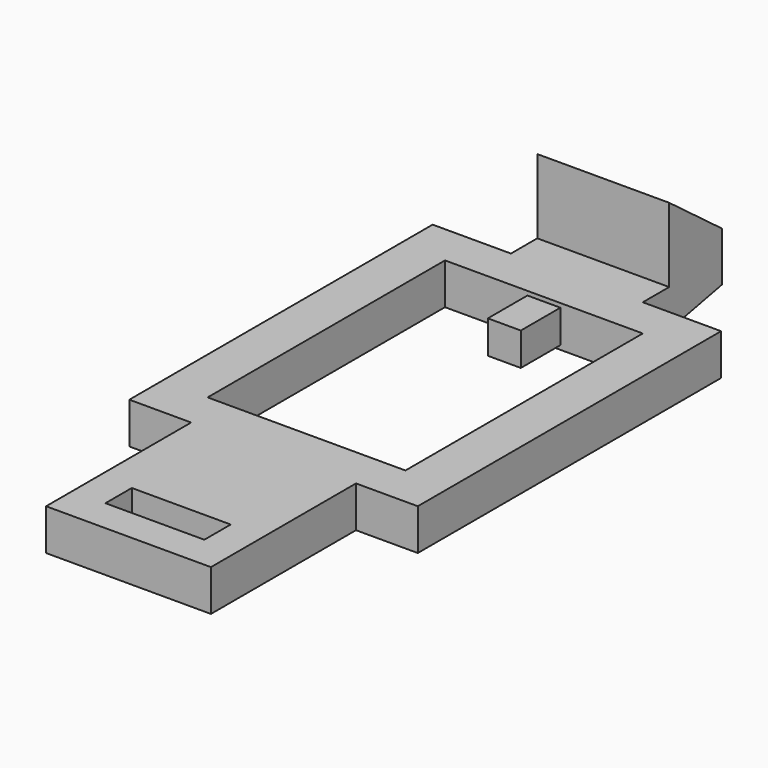
from build123d import *

# Parameters (mm, degrees)
F0_W     = 6
F0_H     = 2
F1_DEPTH = 2.5
F2_W     = 8
F2_H     = 4
F3_DEPTH = 4.5
F4_SIZE2 = 3.99999
F4_SIZE  = 2.99999
F5_SIZE2 = 1
F5_SIZE  = 5
F6_W     = 2
F6_H     = 3
F7_DEPTH = 0.25
F8_W     = 2
F8_H     = 3
F9_DEPTH = 0.25


# Not quite as in the source:
# - a fillet or chamfer is up to 0.001 mm smaller than in the source, because OpenCascade refuses the exact size


with BuildPart() as f1:
    # F0 (on Top) → F1 (new body)
    with BuildSketch(Plane.XY):
        Polygon((-5, 11), (-5, 0), (5, 0), (5, 11), (8.75, 11), (8.75, 34), (4, 34), (4, 40), (-4, 40), (-4, 34), (-8.75, 34), (-8.75, 11), align=None)
        with Locations((0, 3)):
            Rectangle(F0_W, F0_H, mode=Mode.SUBTRACT)
        Polygon((-6, 13.5), (-6, 31.5), (-1, 31.5), (-1, 28.5), (1, 28.5), (1, 31.5), (6, 31.5), (6, 13.5), align=None, mode=Mode.SUBTRACT)
    extrude(amount=F1_DEPTH)

    # F2 (on face) → F3 (join)
    with BuildSketch(Plane.XY.offset(2.5)):
        with Locations((0, 38)):
            Rectangle(F2_W, F2_H)
    extrude(amount=F3_DEPTH)

    # F4 (size 3 and 4 in the source; OpenCascade refuses exactly that, so slightly less here)
    f4_edges = [f1.edges().sort_by_distance(p)[0] for p in [
        (0, 40, 7),
    ]]
    f4_side = f1.faces().sort_by_distance((0, 40, 3.5))[0]
    chamfer(f4_edges, length=F4_SIZE, length2=F4_SIZE2, reference=f4_side)

    # F5
    f5_edges = [f1.edges().sort_by_distance(p)[0] for p in [
        (0, 40, 0),
    ]]
    f5_side = f1.faces().sort_by_distance((-4.563394, 5.5, 0))[0]
    chamfer(f5_edges, length=F5_SIZE, length2=F5_SIZE2, reference=f5_side)

    # F6 (on face) → F7 (cut)
    with BuildSketch(Plane.XY.offset(2.5)):
        with Locations((0, 30)):
            Rectangle(F6_W, F6_H)
    extrude(amount=-F7_DEPTH, mode=Mode.SUBTRACT)

    # F8 (on face) → F9 (cut)
    with BuildSketch(Plane(origin=(0, 0, 0), x_dir=(1, 0, 0), z_dir=(0, 0, -1))):
        with Locations((0, -30)):
            Rectangle(F8_W, F8_H)
    extrude(amount=-F9_DEPTH, mode=Mode.SUBTRACT)


solid = f1.part
